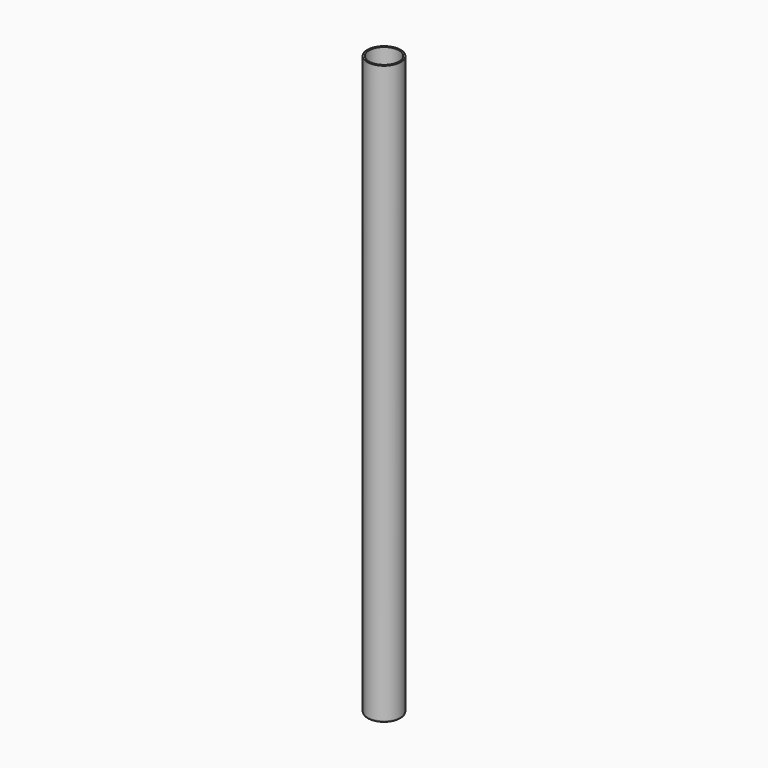
from build123d import *

# Parameters (mm, degrees)
F0_R     = 9
F1_DEPTH = 345
F2_T     = 1


# Not quite as in the source:
# - a fillet or chamfer that OpenCascade refuses, or shapes differently, is made with other operations: its cross-section is extruded or revolved along the edge and cut away or added


with BuildPart() as f1:
    # F0 (on Top) → F1 (new body)
    with BuildSketch(Plane.XY):
        Circle(F0_R)
    extrude(amount=-F1_DEPTH)

    # F2
    f2_openings = [f1.faces().sort_by_distance(p)[0] for p in [
        (0, 0, 0),
    ]]
    offset(amount=F2_T, openings=f2_openings, kind=Kind.INTERSECTION)

    # F3: fillet of radius 1 on 1 edges, made by hand

    # F3_s1 → F3_t2 (revolve, cut)
    with BuildSketch(Plane.XZ):
        with BuildLine():
            ThreePointArc((10, -345), (9.7071067812, -345.7071067812), (9, -346))
            Line((9, -346), (10, -346))
            Line((10, -346), (10, -345))
        make_face()
    revolve(axis=Axis((0, 0, -346), (0, 0, 1)), mode=Mode.SUBTRACT)


solid = f1.part
